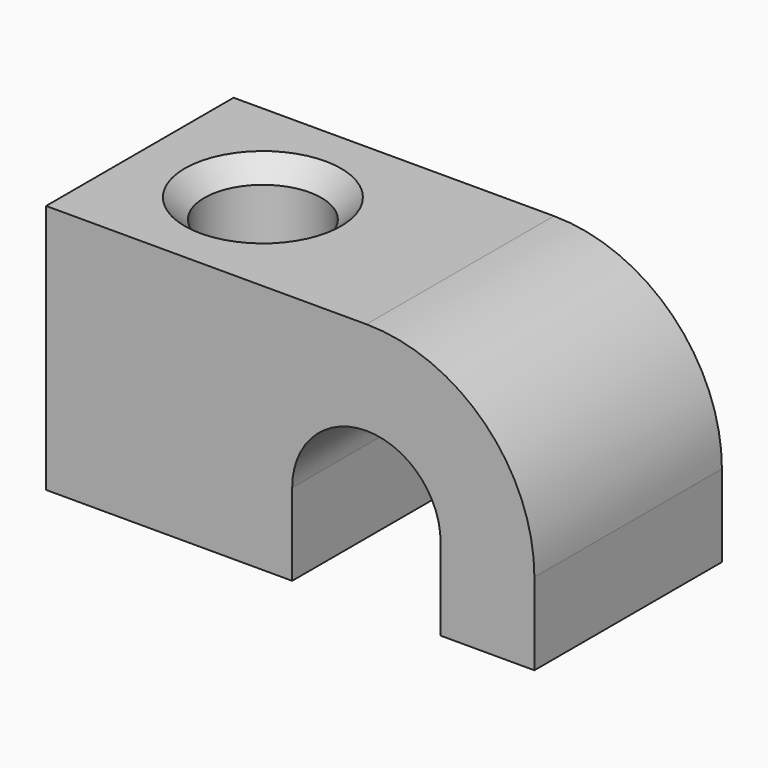
from build123d import *

# Parameters (mm, degrees)
F1_DEPTH       = 6
F3_D           = 3
F3_CSINK_D     = 4
F3_CSINK_ANGLE = 90


# Not quite as in the source:
# - a feature names something its author has since deleted; it is built from what else it names


with BuildPart() as f1:
    # F0 (on Front) → F1 (new body)
    with BuildSketch(Plane.XZ):
        with BuildLine():
            Line((12.5, -2.1), (12.5, 0))
            ThreePointArc((12.5, 0), (11.2405591591, 3.0405591591), (8.2, 4.3))
            Line((8.2, 4.3), (0, 4.3))
            Line((0, 4.3), (0, -2.1))
            Line((0, -2.1), (6.3, -2.1))
            Line((6.3, -2.1), (6.3, 0))
            ThreePointArc((6.3, 0), (8.2, 1.9), (10.1, 0))
            Line((10.1, 0), (10.1, -2.1))
            Line((10.1, -2.1), (12.5, -2.1))
        make_face()
    extrude(amount=F1_DEPTH)

    # F3 (through all)
    with Locations(Plane.XY.offset(4.3)):
        with Locations((3.15, -3)):
            CounterSinkHole(F3_D / 2, F3_CSINK_D / 2, counter_sink_angle=F3_CSINK_ANGLE)


solid = f1.part
